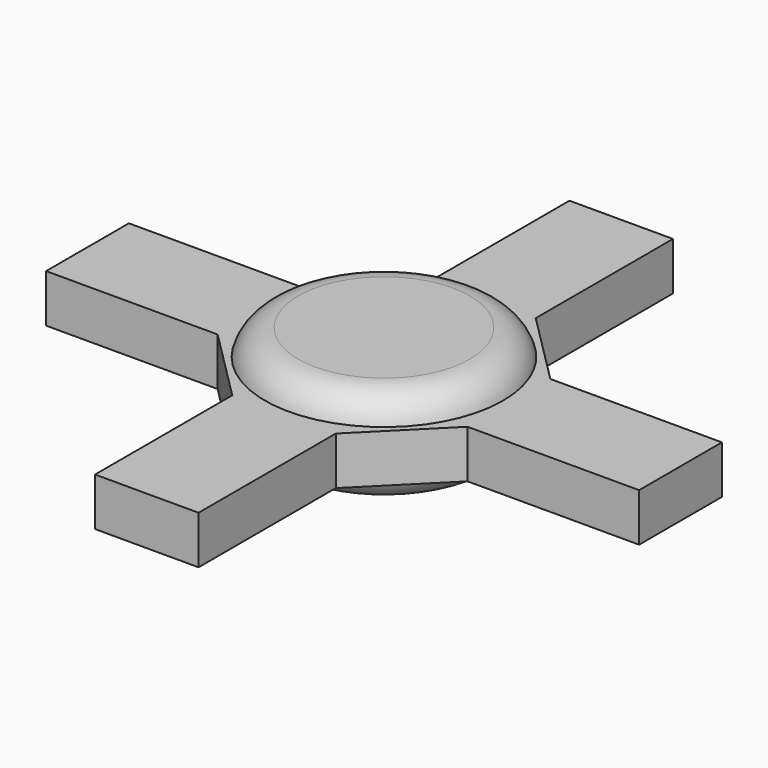
from build123d import *

# Parameters (mm, degrees)
F1_DEPTH = 7.112
F2_DEPTH = 25.4
F3_DEPTH = 25.4
F4_DEPTH = 25.4
F5_DEPTH = 25.4
F6_R     = 17.6209063201
F7_DEPTH = 10.922
F8_DEPTH = 3.556


# Not quite as in the source:
# - a fillet or chamfer that OpenCascade refuses, or shapes differently, is made with other operations: its cross-section is extruded or revolved along the edge and cut away or added


with BuildPart() as f1:
    # F0 (on Top) → F1 (new body)
    with BuildSketch(Plane.XY):
        Polygon((7.6623515216, 18.4985529631), (-7.6623515216, 18.4985529631), (-18.4985529631, 7.6623515216), (-18.4985529631, -7.6623515216), (-7.6623515216, -18.4985529631), (7.6623515216, -18.4985529631), (18.4985529631, -7.6623515216), (18.4985529631, 7.6623515216), align=None)
    extrude(amount=F1_DEPTH)

    # F2 (add): a face of the model
    f2_faces = [f1.faces().sort_by_distance(p)[0] for p in [
        (0, -18.4985529631, 3.556),
    ]]
    extrude(f2_faces, amount=F2_DEPTH)

    # F3 (add): a face of the model
    f3_faces = [f1.faces().sort_by_distance(p)[0] for p in [
        (-18.4985529631, 0, 3.556),
    ]]
    extrude(f3_faces, amount=F3_DEPTH)

    # F4 (add): a face of the model
    f4_faces = [f1.faces().sort_by_distance(p)[0] for p in [
        (0, 18.4985529631, 3.556),
    ]]
    extrude(f4_faces, amount=F4_DEPTH)

    # F5 (add): a face of the model
    f5_faces = [f1.faces().sort_by_distance(p)[0] for p in [
        (18.4985529631, 0, 3.556),
    ]]
    extrude(f5_faces, amount=F5_DEPTH)

    # F6 (on Top) → F7 (join)
    with BuildSketch(Plane.XY):
        Circle(F6_R)
    extrude(amount=F7_DEPTH)

    # F6 (on Top) → F8 (join)
    with BuildSketch(Plane.XY):
        Circle(F6_R)
    extrude(amount=-F8_DEPTH)

    # F9: fillet of radius 5.08 on 1 edges, made by hand

    # F9_s1 → F9_t2 (revolve, cut)
    with BuildSketch(Plane.XZ):
        with BuildLine():
            ThreePointArc((17.6209063201, 7.112), (15.8130694437, 9.8580926284), (12.7022174704, 10.922))
            Line((12.7022174704, 10.922), (17.6209063201, 10.922))
            Line((17.6209063201, 10.922), (17.6209063201, 7.112))
        make_face()
    revolve(axis=Axis((0, 0, 10.922), (0, 0, 1)), mode=Mode.SUBTRACT)

    # F10: fillet of radius 5.08 on 1 edges, made by hand

    # F10_s1 → F10_t2 (revolve, cut)
    with BuildSketch(Plane.XZ):
        with BuildLine():
            ThreePointArc((17.6209063201, 0), (15.7802637067, -2.5716269361), (12.7748951769, -3.556))
            Line((12.7748951769, -3.556), (17.6209063201, -3.556))
            Line((17.6209063201, -3.556), (17.6209063201, 0))
        make_face()
    revolve(axis=Axis((0, 0, -3.556), (0, 0, 1)), mode=Mode.SUBTRACT)


solid = f1.part
